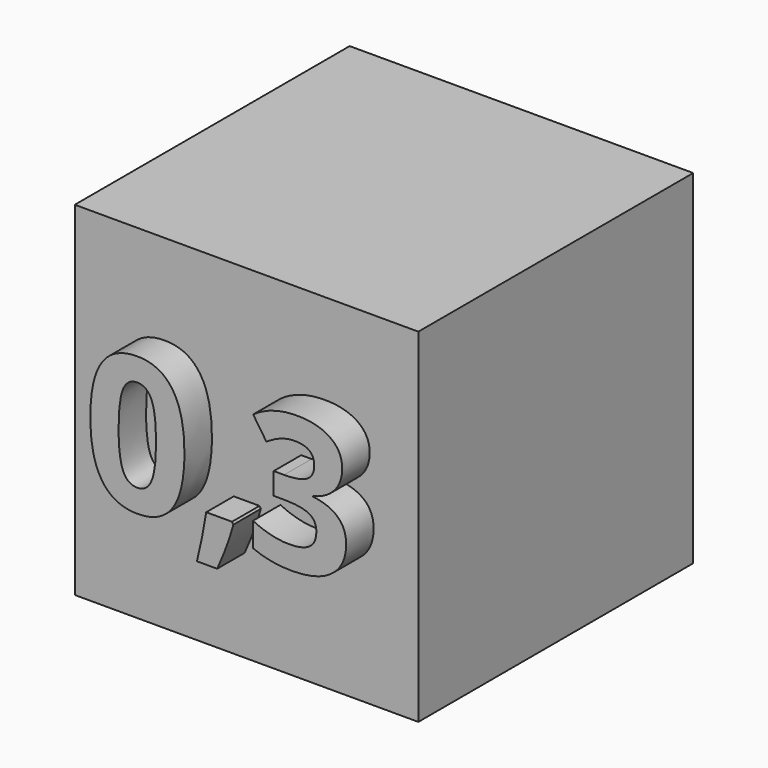
from build123d import *

# Parameters (mm, degrees)
F0_W         = 20
F0_H         = 20
F1_DEPTH     = 20
F2_TEXT_SIZE = 10.974591391
F3_DEPTH     = 2


# Not quite as in the source:
# - Text() gives the source's letters only with a copy of the font that has no kerning and outlines rounded to 1/6400 em; it was checked with that copy


with BuildPart() as f1:
    # F0 (on Front) → F1 (new body)
    with BuildSketch(Plane.XZ):
        with Locations((-10, 10)):
            Rectangle(F0_W, F0_H)
    extrude(amount=F1_DEPTH)

    # F2 (on face) → F3 (join)
    with BuildSketch(Plane.XZ.offset(20)):
        with Locations((-17.8915136494, 6.7885452881)):
            Text('0,3', F2_TEXT_SIZE, font='Open Sans', font_style=FontStyle.BOLD, text_align=(TextAlign.LEFT, TextAlign.BOTTOM))
    extrude(amount=F3_DEPTH)


solid = f1.part
